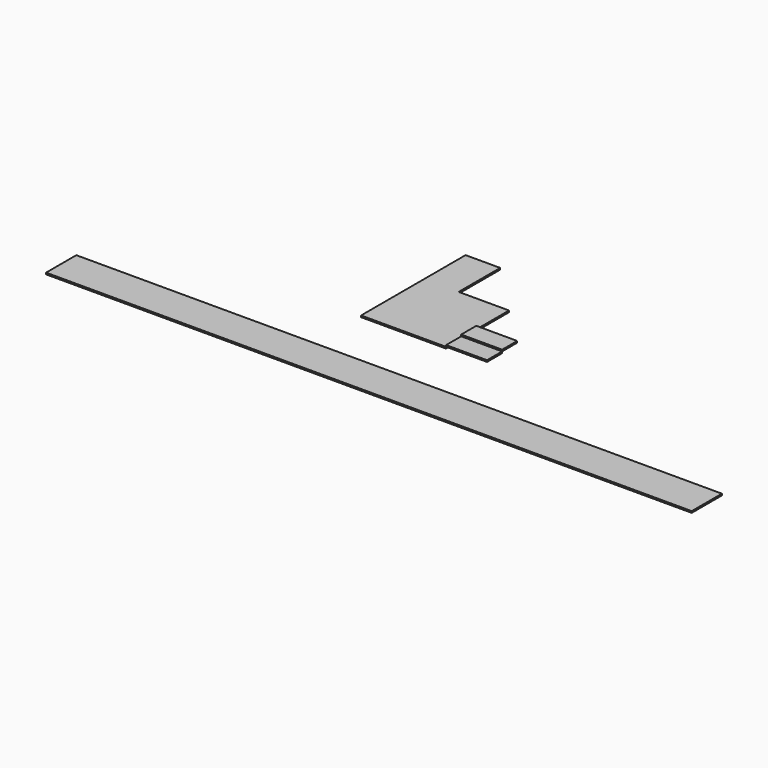
from build123d import *

# Parameters (mm, degrees)
F0_W     = 812.8
F0_H     = 1270
F1_DEPTH = 25.4
F2_W     = 660.4
F2_H     = 304.8
F3_DEPTH = 25.4
F4_W     = 10419.1197770573
F4_H     = 609.6
F5_DEPTH = 25.4
F7_DEPTH = 25.4


# Not quite as in the source:
# - a feature names something its author has since deleted; it is built from what else it names


with BuildPart() as f1:
    # F0 (on Top) → F1 (new body)
    with BuildSketch(Plane.XY):
        Polygon((-1371.6, 0), (-812.8, 0), (-812.8, 1270), (-812.8, 2108.2), (-1371.6, 2108.2), align=None)
        with Locations((-406.4, 635)):
            Rectangle(F0_W, F0_H)
    extrude(amount=F1_DEPTH)


with BuildPart() as f3:
    # F2 (on face) → F3 (new body)
    with BuildSketch(Plane.XY.offset(25.4)):
        with Locations((330.835, 152.4)):
            Rectangle(F2_W, F2_H)
    extrude(amount=F3_DEPTH)


with BuildPart() as f5:
    # F4 (on face) → F5 (new body)
    with BuildSketch(Plane.XY.offset(25.4)):
        with Locations((38.7099906802, -1300.48)):
            Rectangle(F4_W, F4_H)
    extrude(amount=F5_DEPTH)


with BuildPart() as f7:
    # F6 (on face) → F7 (new body)
    with BuildSketch(Plane.XY.offset(50.8)):
        Polygon((0.635, 304.8), (661.035, 304.8), (661.035, 609.6), (0, 609.6), (0, 304.8), align=None)
    extrude(amount=F7_DEPTH)


solid = Compound([f1.part, f3.part, f5.part, f7.part])
